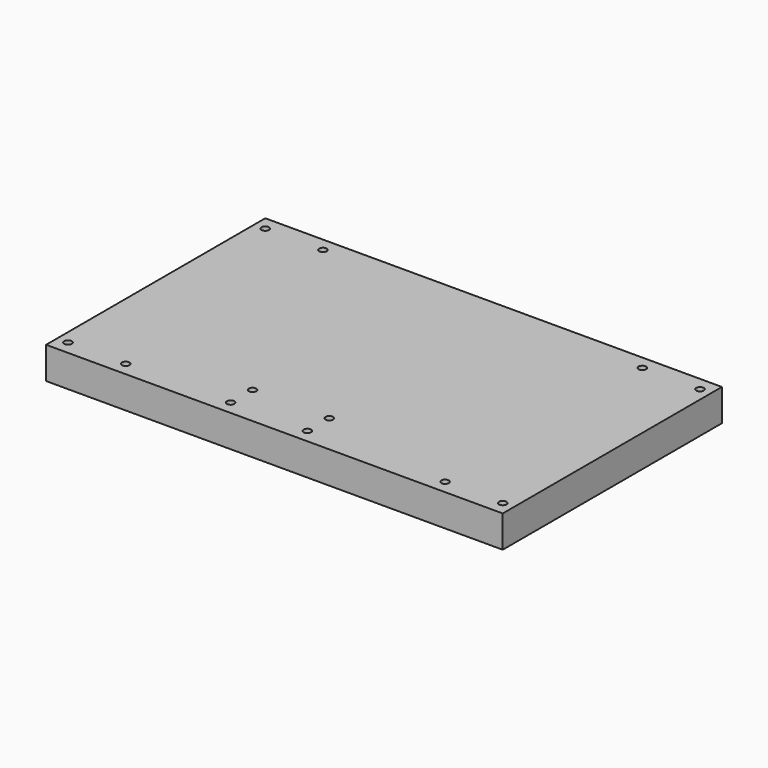
from build123d import *

# Parameters (mm, degrees)
F0_W     = 250
F0_H     = 150
F1_DEPTH = 17.5
F3_D     = 4.1


# Not quite as in the source:
# - the program builds the solid bodies; features that only make, move or delete a surface that nothing else refers to are left out


with BuildPart() as f1:
    # F0 (on Top) → F1 (new body)
    with BuildSketch(Plane.XY):
        with Locations((45.0563491821, 32.5613047183)):
            Rectangle(F0_W, F0_H)
    extrude(amount=F1_DEPTH)

    # F3 (through all)
    with Locations(Plane.XY.offset(17.5)):
        with Locations((-73.9436508179, 100.0613047183), (-42.3736508179, 100.0613047183), (132.4863491821, 100.0613047183), (164.0563491821, 100.0613047183), (164.0563491821, -34.9386952817), (132.4863491821, -34.9386952817), (57.0981395915, -19.9386952817), (57.0981395915, -34.9386952817), (15.0981395915, -19.9386952817), (15.0981395915, -34.9386952817), (-42.3736508179, -34.9386952817), (-73.9436508179, -34.9386952817)):
            Hole(F3_D / 2)


solid = f1.part
